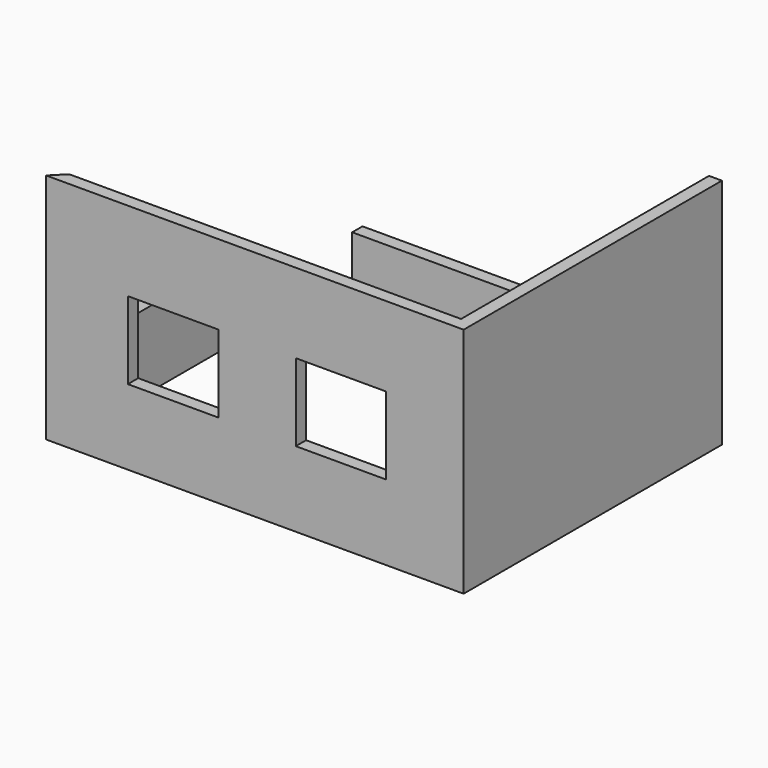
from build123d import *

# Parameters (mm, degrees)
F1_DEPTH  = 889
F3_DEPTH  = 2159
F4_W      = 762
F4_H      = 152.4
F4_W_2    = 914.4
F5_DEPTH  = 2159
F6_W      = 152.4
F6_H      = 1244.6
F7_DEPTH  = 1066.8
F8_W      = 152.4
F8_H      = 1244.6
F9_DEPTH  = 1066.8
F10_DEPTH = 304.8


with BuildPart() as f1:
    # F0 (on Top) → F1 (new body)
    with BuildSketch(Plane.XY):
        Polygon((-1778, 1752.6), (2311.4, 1752.6), (2311.4, -1752.6), (-2311.4, -1752.6), (-2311.4, 609.6), (-2463.8, 609.6), (-2463.8, -1752.6), (-2463.8, -1905), (-2311.4, -1905), (2311.4, -1905), (2463.8, -1905), (2463.8, 1752.6), (2463.8, 1905), (2311.4, 1905), (-1778, 1905), align=None)
    extrude(amount=F1_DEPTH)

    # F2 (on face) → F3 (join)
    with BuildSketch(Plane.XY.offset(889)):
        Polygon((2311.4, 1905), (2311.4, 1752.6), (2311.4, -1752.6), (2311.4, -1905), (2463.8, -1905), (2463.8, 1905), align=None)
    extrude(amount=F3_DEPTH)

    # F4 (on face) → F5 (join)
    with BuildSketch(Plane.XY.offset(889)):
        with Locations((1930.4, -1828.8)):
            Rectangle(F4_W, F4_H)
        with Locations((25.4, -1828.8)):
            Rectangle(F4_W_2, F4_H)
        Polygon((-2463.8, -1905), (-1498.6, -1905), (-1498.6, -1752.6), (-2311.4, -1752.6), align=None)
    extrude(amount=F5_DEPTH)

    # F6 (on face) → F7 (join, through all)
    with BuildSketch(Plane(origin=(1549.4, 0, 0), x_dir=(0, -1, 0), z_dir=(-1, 0, 0))):
        with Locations((1828.8, 2425.7)):
            Rectangle(F6_W, F6_H)
    extrude(amount=F7_DEPTH)

    # F8 (on face) → F9 (join, through all)
    with BuildSketch(Plane(origin=(-431.8, 0, 0), x_dir=(0, -1, 0), z_dir=(-1, 0, 0))):
        with Locations((1828.8, 2425.7)):
            Rectangle(F8_W, F8_H)
    extrude(amount=F9_DEPTH)

    # F10 (cut): a face of the model
    f10_faces = [f1.faces().sort_by_distance(p)[0] for p in [
        (2373.6875121995, 76.2, 3048),
    ]]
    extrude(f10_faces, amount=-F10_DEPTH, mode=Mode.SUBTRACT)


solid = f1.part
